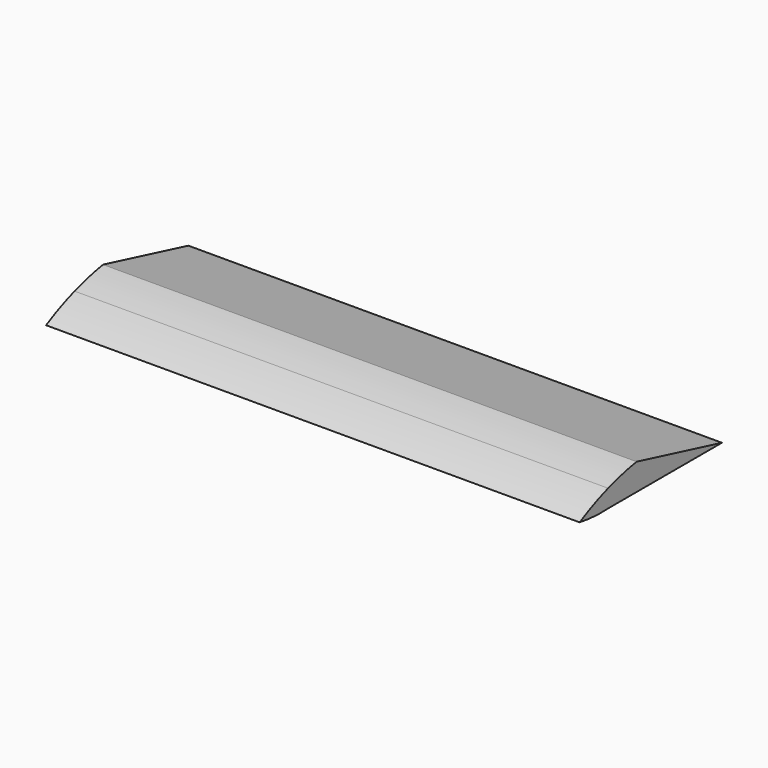
from build123d import *

# Parameters (mm, degrees)
F1_DEPTH = 762


# Not quite as in the source:
# - a feature names something its author has since deleted; it is built from what else it names


with BuildPart() as f1:
    # F0 (on Right) → F1 (new body)
    with BuildSketch(Plane.YZ):
        with BuildLine():
            ThreePointArc((-76.2, 6.35), (-102.0787858137, -3.6681324257), (-127, -15.875))
            ThreePointArc((-127, -15.875), (-101.6930614476, -18.9514831615), (-76.2, -19.05))
            Line((-76.2, -19.05), (-76.2, -17.4625))
            Line((-76.2, -17.4625), (-76.2, 6.35))
        make_face()
        with BuildLine():
            Line((127, -19.05), (-25.4, 19.05))
            ThreePointArc((-25.4, 19.05), (-51.0583154566, 13.7332618264), (-76.2, 6.35))
            Line((-76.2, 6.35), (-76.2, -17.4625))
            Line((-76.2, -17.4625), (-76.2, -19.05))
            Line((-76.2, -19.05), (127, -19.05))
        make_face()
    extrude(amount=F1_DEPTH)


solid = f1.part
